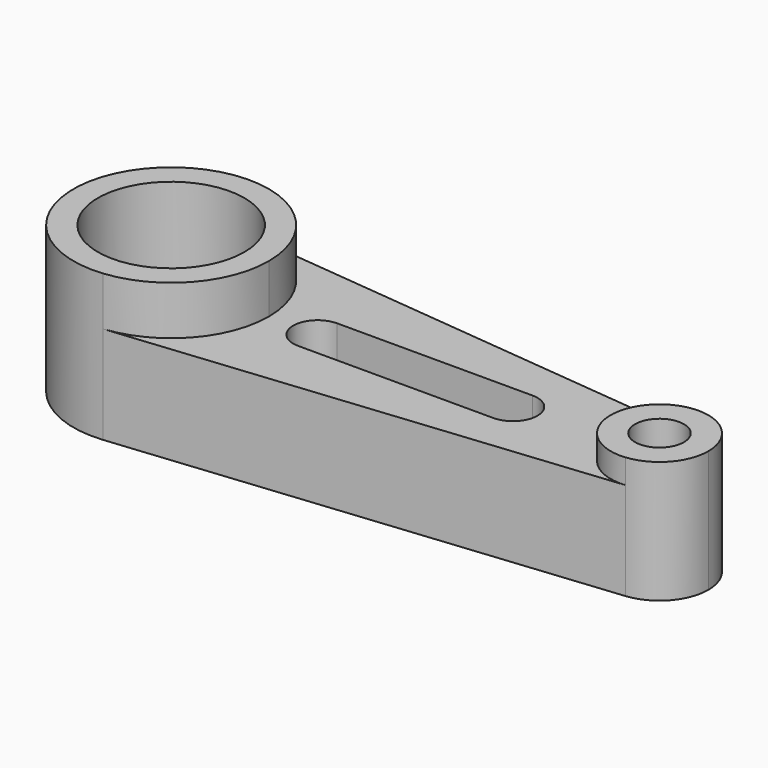
from build123d import *
from build123d import SkipClean  # not in build123d's __all__

# Parameters (mm, degrees)
F0_R     = 19.05
F0_R_2   = 6.35
F1_DEPTH = 38.1
F2_DEPTH = 6.35
F3_DEPTH = 12.7


with BuildPart() as f1:
    # F0 (on Top) → F1 (new body)
    with BuildSketch(Plane.XY):
        with BuildLine():
            ThreePointArc((-35.56, -25.2726809025), (-19.2628558428, -17.0388379885), (-12.7, 0))
            ThreePointArc((-12.7, 0), (-19.2628558428, 17.0388379885), (-35.56, 25.2726809025))
            ThreePointArc((-35.56, 25.2726809025), (-63.5, 0), (-35.56, -25.2726809025))
        make_face()
        with Locations((-38.1, 0)):
            Circle(F0_R, mode=Mode.SUBTRACT)
        with BuildLine():
            ThreePointArc((-35.56, 25.2726809025), (-19.2628558428, 17.0388379885), (-12.7, 0))
            ThreePointArc((-12.7, 0), (-19.2628558428, -17.0388379885), (-35.56, -25.2726809025))
            Line((-35.56, -25.2726809025), (90.17, -12.6363404513))
            ThreePointArc((90.17, -12.6363404513), (76.2, 0), (90.17, 12.6363404513))
            Line((90.17, 12.6363404513), (-35.56, 25.2726809025))
        make_face()
        with BuildLine():
            ThreePointArc((0, -6.35), (-6.35, 0), (0, 6.35))
            Line((0, 6.35), (50.8, 6.35))
            ThreePointArc((50.8, 6.35), (57.15, 0), (50.8, -6.35))
            Line((50.8, -6.35), (0, -6.35))
        make_face(mode=Mode.SUBTRACT)
        with BuildLine():
            ThreePointArc((101.6, 0), (98.3185720786, 8.5194189943), (90.17, 12.6363404513))
            ThreePointArc((90.17, 12.6363404513), (76.2, 0), (90.17, -12.6363404513))
            ThreePointArc((90.17, -12.6363404513), (98.3185720786, -8.5194189943), (101.6, 0))
        make_face()
        with Locations((88.9, 0)):
            Circle(F0_R_2, mode=Mode.SUBTRACT)
    extrude(amount=-F1_DEPTH)

    # F0 (on Top) → F2 (cut)
    with BuildSketch(Plane.XY):
        with BuildLine():
            ThreePointArc((101.6, 0), (98.3185720786, 8.5194189943), (90.17, 12.6363404513))
            ThreePointArc((90.17, 12.6363404513), (76.2, 0), (90.17, -12.6363404513))
            ThreePointArc((90.17, -12.6363404513), (98.3185720786, -8.5194189943), (101.6, 0))
        make_face()
        with Locations((88.9, 0)):
            Circle(F0_R_2, mode=Mode.SUBTRACT)
    extrude(amount=-F2_DEPTH, mode=Mode.SUBTRACT)

    # F0 (on Top) → F3 (cut)
    with BuildSketch(Plane.XY):
        with BuildLine():
            ThreePointArc((-35.56, 25.2726809025), (-19.2628558428, 17.0388379885), (-12.7, 0))
            ThreePointArc((-12.7, 0), (-19.2628558428, -17.0388379885), (-35.56, -25.2726809025))
            Line((-35.56, -25.2726809025), (90.17, -12.6363404513))
            ThreePointArc((90.17, -12.6363404513), (76.2, 0), (90.17, 12.6363404513))
            Line((90.17, 12.6363404513), (-35.56, 25.2726809025))
        make_face()
        with BuildLine():
            ThreePointArc((0, -6.35), (-6.35, 0), (0, 6.35))
            Line((0, 6.35), (50.8, 6.35))
            ThreePointArc((50.8, 6.35), (57.15, 0), (50.8, -6.35))
            Line((50.8, -6.35), (0, -6.35))
        make_face(mode=Mode.SUBTRACT)
    with SkipClean():  # cleaning this boolean's faces spoils the solid; the shape is the same uncleaned
        extrude(amount=-F3_DEPTH, mode=Mode.SUBTRACT)


solid = f1.part
